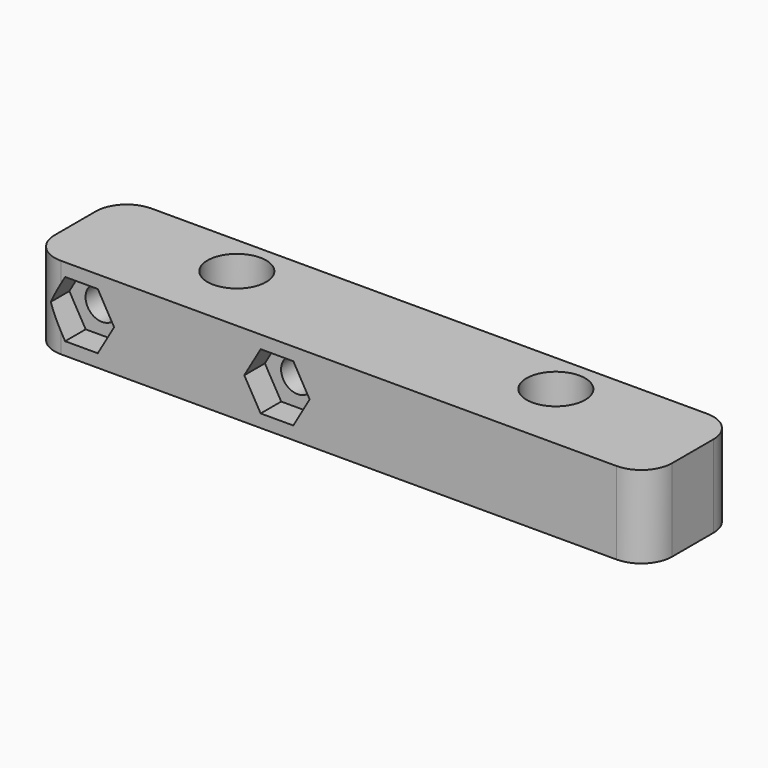
from build123d import *

# Parameters (mm, degrees)
F1_R        = 1.6
F2_DEPTH    = 8
F3_R        = 2.85
F4_DEPTH    = 3
F6_DEPTH    = 2.5
F7_D        = 3.2
F8_T1_DEPTH = 23


# Not quite as in the source:
# - a fillet or chamfer that OpenCascade refuses, or shapes differently, is made with other operations: its cross-section is extruded or revolved along the edge and cut away or added


with BuildPart() as f2:
    # F1 (on Top) → F2 (new body)
    with BuildSketch(Plane.XY):
        Polygon((45.5, -7), (45.5, 0), (45.5, 4), (-14.5, 4), (-14.5, 0), (-14.5, -0.2), (-14.5, -7), (-9.5, -7), (40.5, -7), align=None)
        Circle(F1_R, mode=Mode.SUBTRACT)
        with Locations((31, 0)):
            Circle(F1_R, mode=Mode.SUBTRACT)
    extrude(amount=F2_DEPTH)

    # F3 (on face) → F4 (cut)
    with BuildSketch(Plane.XY.offset(8)):
        Circle(F3_R)
        with Locations((31, 0)):
            Circle(F3_R)
    extrude(amount=-F4_DEPTH, mode=Mode.SUBTRACT)

    # F5 (on face) → F6 (cut)
    with BuildSketch(Plane.XZ.offset(7)):
        Polygon((-7.9122867597, 6.75), (-11.0877132403, 6.75), (-12.6754264805, 4), (-11.0877132403, 1.25), (-7.9122867597, 1.25), (-6.3245735195, 4), align=None)
        Polygon((11.0877132403, 6.75), (7.9122867597, 6.75), (6.3245735195, 4), (7.9122867597, 1.25), (11.0877132403, 1.25), (12.6754264805, 4), align=None)
    extrude(amount=-F6_DEPTH, mode=Mode.SUBTRACT)

    # F7 (through all)
    with Locations(Plane.XZ.offset(7)):
        with Locations((-9.5, 4), (9.5, 4)):
            Hole(F7_D / 2)

    # F8: fillet of radius 3 on 4 edges, made by hand

    # F8_s2 → F8_t1 (cut)
    with BuildSketch(Plane.XY.offset(-7.5)):
        with BuildLine():
            ThreePointArc((-11.5, 4), (-13.6213203436, 3.1213203436), (-14.5, 1))
            Line((-14.5, 1), (-14.5, 4))
            Line((-14.5, 4), (-11.5, 4))
        make_face()
        with BuildLine():
            ThreePointArc((45.5, -4), (44.6213203436, -6.1213203436), (42.5, -7))
            Line((42.5, -7), (45.5, -7))
            Line((45.5, -7), (45.5, -4))
        make_face()
        with BuildLine():
            ThreePointArc((45.5, 1), (44.6213203436, 3.1213203436), (42.5, 4))
            Line((42.5, 4), (45.5, 4))
            Line((45.5, 4), (45.5, 1))
        make_face()
        with BuildLine():
            ThreePointArc((-11.5, -7), (-13.6213203436, -6.1213203436), (-14.5, -4))
            Line((-14.5, -4), (-14.5, -7))
            Line((-14.5, -7), (-11.5, -7))
        make_face()
    extrude(amount=F8_T1_DEPTH, mode=Mode.SUBTRACT)


solid = f2.part
